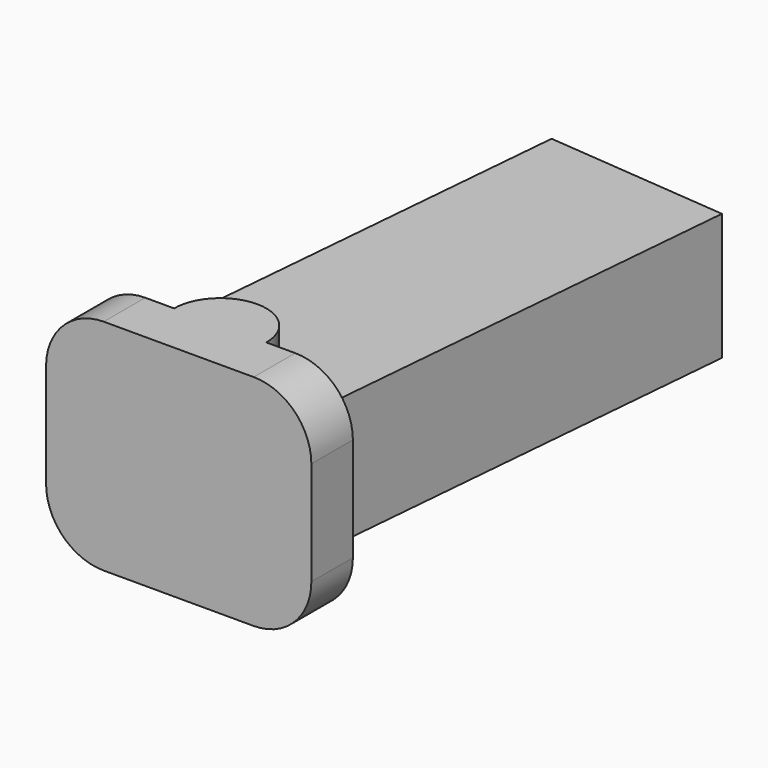
from build123d import *

# Parameters (mm, degrees)
F1_DEPTH  = 5.5
F2_DEPTH  = 9.5
F5_DEPTH  = 4
F7_DEPTH  = 4
F8_R      = 5
F9_R      = 5
F10_R     = 5
F11_R     = 5
F3_W      = 12.9391151695
F3_H      = 8
F12_DEPTH = 40


# Not quite as in the source:
# - a feature names something its author has since deleted; it is built from what else it names


with BuildPart() as f1:
    # F0 (on Top) → F1 (new body, symmetric)
    with BuildSketch(Plane.XY):
        Polygon((45.3994634662, -11.2350502836), (29.5210014421, -9.8458648622), (25.8999169252, -51.2350502836), (41.8999169252, -51.2350502836), align=None)
    extrude(amount=F1_DEPTH, both=True)

    # F0 (on Top) → F2 (join, symmetric)
    with BuildSketch(Plane.XY):
        Polygon((41.8999169252, -51.2350502836), (25.8999169252, -51.2350502836), (22.3999169252, -51.2350502836), (22.3999169252, -55.7350502836), (45.3999169252, -55.7350502836), (45.3999169252, -51.2350502836), align=None)
    extrude(amount=F2_DEPTH, both=True)

    # F4 (on face) → F5 (join)
    with BuildSketch(Plane.XY.offset(5.5)):
        with BuildLine():
            Line((29.8999169252, -51.2350502836), (37.8999169252, -51.2350502836))
            ThreePointArc((37.8999169252, -51.2350502836), (33.8999169252, -47.2350502836), (29.8999169252, -51.2350502836))
        make_face()
    extrude(amount=F5_DEPTH)

    # F6 (on face) → F7 (join)
    with BuildSketch(Plane(origin=(0, 0, -5.5), x_dir=(1, 0, 0), z_dir=(0, 0, -1))):
        with BuildLine():
            ThreePointArc((29.8999169252, 51.2350502836), (33.8999169252, 47.2350502836), (37.8999169252, 51.2350502836))
            Line((37.8999169252, 51.2350502836), (29.8999169252, 51.2350502836))
        make_face()
    extrude(amount=F7_DEPTH)

    # F8
    f8_edges = [f1.edges().sort_by_distance(p)[0] for p in [
        (22.399917, -53.48505, 9.5),
    ]]
    fillet(f8_edges, radius=F8_R)

    # F9
    f9_edges = [f1.edges().sort_by_distance(p)[0] for p in [
        (45.399917, -53.48505, 9.5),
    ]]
    fillet(f9_edges, radius=F9_R)

    # F10
    f10_edges = [f1.edges().sort_by_distance(p)[0] for p in [
        (45.399917, -53.48505, -9.5),
    ]]
    fillet(f10_edges, radius=F10_R)

    # F11
    f11_edges = [f1.edges().sort_by_distance(p)[0] for p in [
        (22.399917, -53.48505, -9.5),
    ]]
    fillet(f11_edges, radius=F11_R)

    # F3 (on face) → F12 (cut)
    with BuildSketch(Plane(origin=(-0.6306130728, -7.2079404052, 0), x_dir=(-0.9961946981, 0.0871557427, 0), z_dir=(0.0871557427, 0.9961946981, 0))):
        with Locations((-38.2363463688, 0)):
            Rectangle(F3_W, F3_H)
    extrude(amount=-F12_DEPTH, mode=Mode.SUBTRACT)


solid = f1.part
